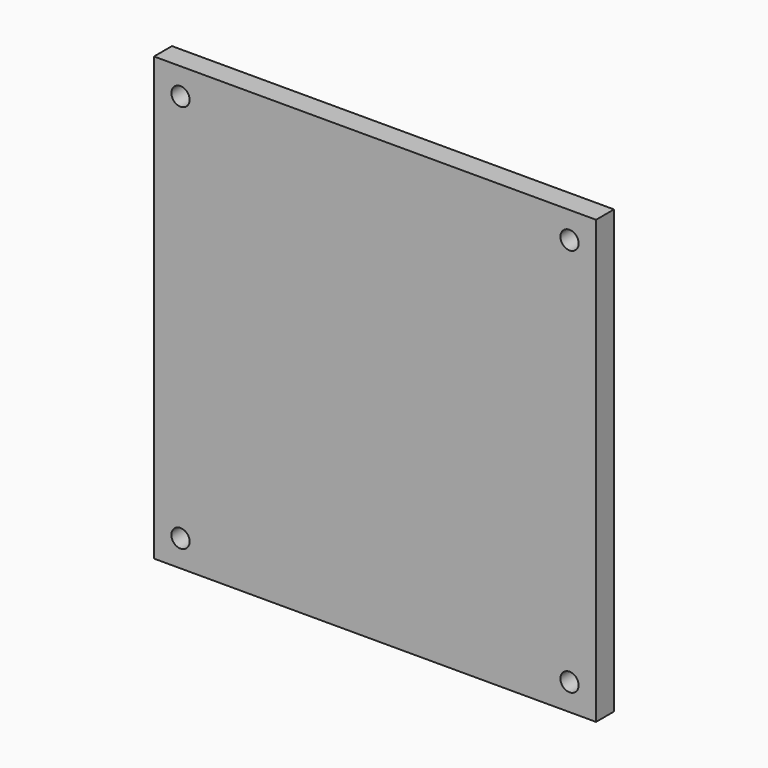
from build123d import *

# Parameters (mm, degrees)
F0_W     = 250
F0_H     = 250
F1_DEPTH = 12.7
F2_D     = 10.3


# Not quite as in the source:
# - a length typed as a fraction of an inch, garbled in the dataset ("3 / 203.2 mm" for 3/8 in), is restored


with BuildPart() as f1:
    # F0 (on Front) → F1 (new body)
    with BuildSketch(Plane.XZ):
        Rectangle(F0_W, F0_H)
    extrude(amount=F1_DEPTH)

    # F2 (through all)
    with Locations(Plane(origin=(0, 0, 0), x_dir=(1, 0, 0), z_dir=(0, 1, 0))):
        with Locations((-110, -110), (-110, 110), (110, 110), (110, -110)):
            Hole(F2_D / 2)


solid = f1.part
